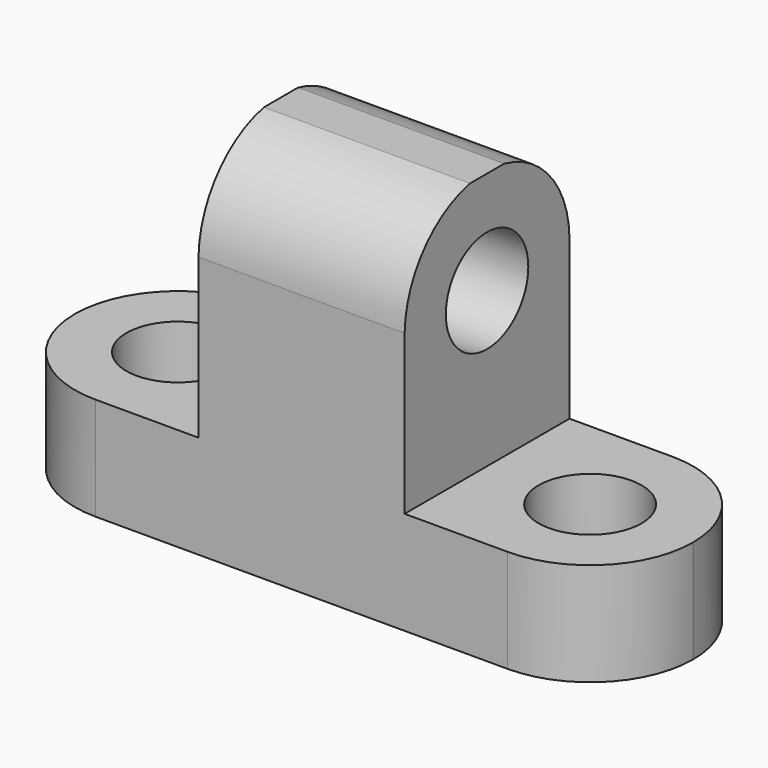
from build123d import *

# Parameters (mm, degrees)
F1_DEPTH = 25.4
F2_R     = 6.35
F3_DEPTH = 25.4
F4_R     = 6.35
F5_DEPTH = 25.4
F6_R     = 6.35
F7_DEPTH = 25.4


# Not quite as in the source:
# - ends of sketch curves that miss each other by under 0.0002 mm in the source are joined


with BuildPart() as f1:
    # F0 (on Front) → F1 (new body)
    with BuildSketch(Plane.XZ):
        Polygon((0, 12.7), (0, 0), (76.2, 0), (76.2, 12.7), (50.8, 12.7), (50.8, 44.45), (25.4, 44.45), (25.4, 12.7), align=None)
    extrude(amount=F1_DEPTH)

    # F2 (on face) → F3 (cut)
    with BuildSketch(Plane.YZ.offset(50.8)):
        with BuildLine():
            ThreePointArc((-25.4, 32.294421317), (-22.4820111245, 40.1263057346), (-15.3294772723, 44.45))
            Line((-15.3294772723, 44.45), (-25.4, 44.45))
            Line((-25.4, 44.45), (-25.4, 32.294421317))
        make_face()
        with BuildLine():
            ThreePointArc((-10.0705227277, 44.45), (-2.9179888755, 40.1263057346), (0, 32.294421317))
            Line((0, 32.294421317), (0, 44.45))
            Line((0, 44.45), (-10.0705227277, 44.45))
        make_face()
        with Locations((-12.7, 31.75)):
            Circle(F2_R)
    extrude(amount=-F3_DEPTH, mode=Mode.SUBTRACT)

    # F4 (on face) → F5 (cut)
    with BuildSketch(Plane.XY.offset(12.7)):
        with BuildLine():
            ThreePointArc((63.5, -3.1832e-06), (72.4802600435, -3.7197427535), (76.2000063664, -12.7))
            Line((76.2000063664, -12.7), (76.2, 0))
            Line((76.2, 0), (63.5, -3.1832e-06))
        make_face()
        with BuildLine():
            ThreePointArc((76.2000063664, -12.7), (72.4802600435, -21.6802572465), (63.5, -25.3999968168))
            Line((63.5, -25.3999968168), (76.2, -25.4))
            Line((76.2, -25.4), (76.2000063664, -12.7))
        make_face()
        with Locations((63.5, -12.7)):
            Circle(F4_R)
    extrude(amount=-F5_DEPTH, mode=Mode.SUBTRACT)

    # F6 (on face) → F7 (cut)
    with BuildSketch(Plane.XY.offset(12.7)):
        with Locations((12.7, -12.7)):
            Circle(F6_R)
        with BuildLine():
            ThreePointArc((0, -12.7), (3.7197438789, -3.7197438789), (12.7, 0))
            Line((12.7, 0), (0, 0))
            Line((0, 0), (0, -12.7))
        make_face()
        with BuildLine():
            ThreePointArc((12.7, -25.4), (3.7197438789, -21.6802561211), (0, -12.7))
            Line((0, -12.7), (0, -25.4))
            Line((0, -25.4), (12.7, -25.4))
        make_face()
    extrude(amount=-F7_DEPTH, mode=Mode.SUBTRACT)


solid = f1.part
